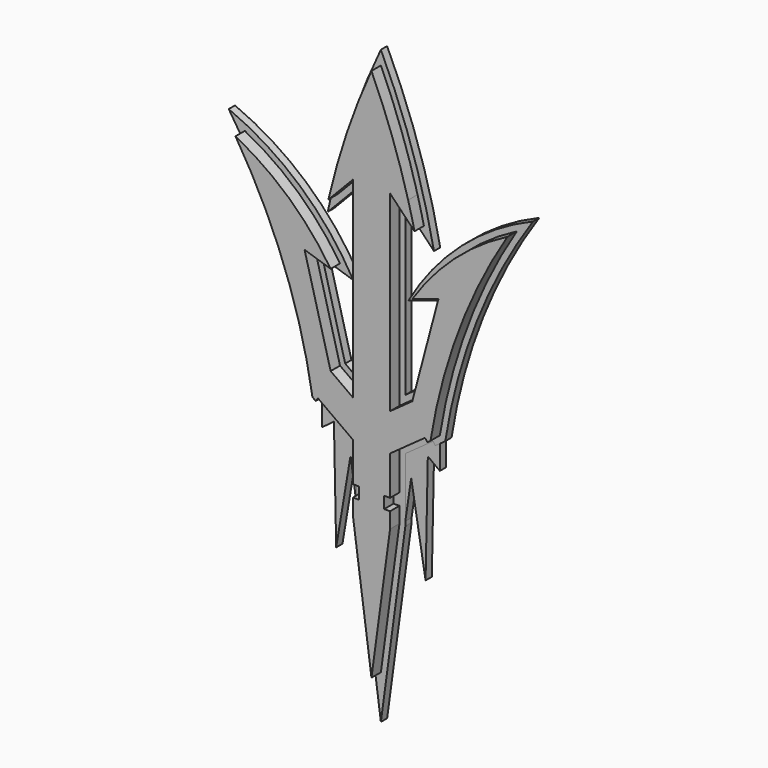
from build123d import *

# Parameters (mm, degrees)
F0_W     = 9.5
F0_H     = 3
F0_W_2   = 4.75
F0_H_2   = 6.5
F0_W_3   = 6.5
F1_DEPTH = 5
F3_DEPTH = 2
F5_DEPTH = 2


with BuildPart() as f1:
    # F0 (on Front) → F1 (new body)
    with BuildSketch(Plane.XZ):
        Polygon((4.75, -32.75), (4.75, -31.75), (0, -31.75), (-4.75, -31.75), (-4.75, -32.75), align=None)
        Polygon((0, -31.75), (4.75, -31.75), (4.75, -26.75), (4.75, -17.25), (4.75, 25.25), (0, 25.25), (-4.75, 25.25), (-4.75, -17.25), (-4.75, -26.75), (-4.75, -31.75), align=None)
        with BuildLine():
            Line((4.75, -17.25), (4.75, -26.75))
            Line((4.75, -26.75), (13.6785707143, -20.325))
            Line((13.6785707143, -20.325), (14.2626616234, -21.1366882468))
            Line((14.2626616234, -21.1366882468), (15.0743498701, -20.5525973377))
            ThreePointArc((15.0743498701, -20.5525973377), (22.2760836347, 6.5903692937), (34.75, 31.75))
            ThreePointArc((34.75, 31.75), (21.1663739273, 22.3753288761), (10.4318177273, 9.8386363636))
            Line((10.4318177273, 9.8386363636), (17.0997445143, 11.9690711462))
            Line((17.0997445143, 11.9690711462), (10.4318177273, -13.1613636364))
            Line((10.4318177273, -13.1613636364), (4.75, -17.25))
        make_face()
        with Locations((0, -34.25)):
            Rectangle(F0_W, F0_H)
        Polygon((4.75, -36.75), (4.75, -35.75), (-4.75, -35.75), (-4.75, -36.75), (-3.25, -36.75), (3.25, -36.75), align=None)
        with BuildLine():
            Line((-13.6785707143, -20.325), (-4.75, -26.75))
            Line((-4.75, -26.75), (-4.75, -17.25))
            Line((-4.75, -17.25), (-10.4318177273, -13.1613636364))
            Line((-10.4318177273, -13.1613636364), (-17.0997445143, 11.9690711462))
            Line((-17.0997445143, 11.9690711462), (-10.4318177273, 9.8386363636))
            ThreePointArc((-10.4318177273, 9.8386363636), (-21.1663739273, 22.3753288761), (-34.75, 31.75))
            ThreePointArc((-34.75, 31.75), (-22.2760836347, 6.5903692937), (-15.0743498701, -20.5525973377))
            Line((-15.0743498701, -20.5525973377), (-14.2626616234, -21.1366882468))
            Line((-14.2626616234, -21.1366882468), (-13.6785707143, -20.325))
        make_face()
        with Locations((2.375, 28.5)):
            Rectangle(F0_W_2, F0_H_2)
        Polygon((8.8, 31.75), (4.75, 31.75), (11, 25.25), align=None)
        Polygon((0, 31.75), (4.75, 31.75), (8.8, 31.75), (0, 57.75), align=None)
        with Locations((-2.375, 28.5)):
            Rectangle(F0_W_2, F0_H_2)
        with BuildLine():
            Line((8.8, 31.75), (11, 25.25))
            ThreePointArc((11, 25.25), (10.2159514871, 28.5079487405), (9.3685639152, 31.75))
            Line((9.3685639152, 31.75), (8.8, 31.75))
        make_face()
        with Locations((0, -38.25)):
            Rectangle(F0_W_3, F0_H)
        Polygon((-4.75, 31.75), (0, 31.75), (0, 57.75), (-11, 25.25), align=None)
        with BuildLine():
            Line((0, 57.75), (8.8, 31.75))
            Line((8.8, 31.75), (9.3685639152, 31.75))
            ThreePointArc((9.3685639152, 31.75), (5.207479083, 44.9385232965), (0, 57.75))
        make_face()
        Polygon((4.75, -39.75), (3.25, -39.75), (-3.25, -39.75), (-4.75, -39.75), (-4.75, -40.75), (4.75, -40.75), align=None)
        with BuildLine():
            ThreePointArc((0, 57.75), (-6.3126627605, 41.7750550882), (-11, 25.25))
            Line((-11, 25.25), (0, 57.75))
        make_face()
        Polygon((4.75, -43.75), (4.75, -40.75), (-4.75, -40.75), (-4.75, -43.75), (0, -43.75), align=None)
        Polygon((0, -78.75), (4.75, -43.75), (0, -43.75), align=None)
        Polygon((0, -43.75), (-4.75, -43.75), (0, -78.75), align=None)
    extrude(amount=F1_DEPTH)


with BuildPart() as f3:
    # F2 (on face) → F3 (new body)
    with BuildSketch(Plane(origin=(0, 0, 0), x_dir=(-1, 0, 0), z_dir=(0, 1, 0))):
        Polygon((15.0743498701, -28.5525973377), (15.0743498701, -20.5525973377), (14.2626616234, -21.1366882468), (13.6785707143, -20.325), (4.75, -26.75), (4.75, -36.75), (3.25, -36.75), (3.25, -39.75), (4.75, -39.75), (4.75, -43.75), (0, -78.75), (1, -78.75), (7.7438349836, -32.4999243021), (11.4220166579, -54.3695688248), (11.9964974001, -26.2390598655), align=None)
    extrude(amount=-F3_DEPTH)


with BuildPart() as f3b:
    # F2 (on face) → F3, piece 2 (new body)
    with BuildSketch(Plane(origin=(0, 0, 0), x_dir=(-1, 0, 0), z_dir=(0, 1, 0))):
        Polygon((-1, -78.75), (0, -78.75), (-4.75, -43.75), (-4.75, -39.75), (-3.25, -39.75), (-3.25, -36.75), (-4.75, -36.75), (-4.75, -26.75), (-13.6785707143, -20.325), (-14.2626616234, -21.1366882468), (-15.0743498701, -20.5525973377), (-15.0743498701, -28.5525973377), (-11.9964974001, -26.2390598655), (-11.4220166579, -54.3695688248), (-7.7438349836, -32.4999243021), align=None)
    extrude(amount=-F3_DEPTH)


with BuildPart() as f5:
    # F4 (on face) → F5 (new body)
    with BuildSketch(Plane(origin=(0, 0, 0), x_dir=(-1, 0, 0), z_dir=(0, 1, 0))):
        with BuildLine():
            Line((9.1197276527, -12.2575435817), (6.25, -14.3225997658))
            Line((6.25, -14.3225997658), (6.25, 28.0258373444))
            Line((6.25, 28.0258373444), (13.5709714754, 20.4120270099))
            ThreePointArc((13.5709714754, 20.4120270099), (8.0601511253, 41.2813035717), (0, 61.3045353033))
            ThreePointArc((0, 61.3045353033), (-8.0601511253, 41.2813035717), (-13.5709714754, 20.4120270099))
            Line((-13.5709714754, 20.4120270099), (-6.25, 28.0258373444))
            Line((-6.25, 28.0258373444), (-6.25, -14.3225997658))
            Line((-6.25, -14.3225997658), (-9.1197276527, -12.2575435817))
            Line((-9.1197276527, -12.2575435817), (-14.9475706012, 9.7067388435))
            Line((-14.9475706012, 9.7067388435), (-7.0573343808, 7.185770299))
            ThreePointArc((-7.0573343808, 7.185770299), (-20.623685191, 23.9014967836), (-38.8766030738, 35.3160653244))
            ThreePointArc((-38.8766030738, 35.3160653244), (-24.5064831966, 8.2050547659), (-16.4583681212, -21.4046578724))
            Line((-16.4583681212, -21.4046578724), (-13.9212656169, -23.2303569805))
            Line((-13.9212656169, -23.2303569805), (-13.3371747078, -22.4186687338))
            Line((-13.3371747078, -22.4186687338), (-6.25, -27.5186000615))
            Line((-6.25, -27.5186000615), (-6.25, -38.25))
            Line((-6.25, -38.25), (-6.25, -43.8513212997))
            Line((-6.25, -43.8513212997), (0, -89.9039528787))
            Line((0, -89.9039528787), (6.25, -43.8513212997))
            Line((6.25, -43.8513212997), (6.25, -38.25))
            Line((6.25, -38.25), (6.25, -27.5186000615))
            Line((6.25, -27.5186000615), (13.3371747078, -22.4186687338))
            Line((13.3371747078, -22.4186687338), (13.9212656169, -23.2303569805))
            Line((13.9212656169, -23.2303569805), (16.4583681212, -21.4046578724))
            ThreePointArc((16.4583681212, -21.4046578724), (24.5064831966, 8.2050547659), (38.8766030738, 35.3160653244))
            ThreePointArc((38.8766030738, 35.3160653244), (20.623685191, 23.9014967836), (7.0573343808, 7.185770299))
            Line((7.0573343808, 7.185770299), (14.9475706012, 9.7067388435))
            Line((14.9475706012, 9.7067388435), (9.1197276527, -12.2575435817))
        make_face()
        with BuildLine():
            Line((-4.75, -26.75), (-13.6785707143, -20.325))
            Line((-13.6785707143, -20.325), (-14.2626616234, -21.1366882468))
            Line((-14.2626616234, -21.1366882468), (-15.0743498701, -20.5525973377))
            ThreePointArc((-15.0743498701, -20.5525973377), (-22.2760836347, 6.5903692937), (-34.75, 31.75))
            ThreePointArc((-34.75, 31.75), (-21.1663739273, 22.3753288761), (-10.4318177273, 9.8386363636))
            Line((-10.4318177273, 9.8386363636), (-17.0997445143, 11.9690711462))
            Line((-17.0997445143, 11.9690711462), (-10.4318177273, -13.1613636364))
            Line((-10.4318177273, -13.1613636364), (-4.75, -17.25))
            Line((-4.75, -17.25), (-4.75, 31.75))
            Line((-4.75, 31.75), (-11, 25.25))
            ThreePointArc((-11, 25.25), (-6.3126627605, 41.7750550882), (0, 57.75))
            ThreePointArc((0, 57.75), (6.3126627605, 41.7750550882), (11, 25.25))
            Line((11, 25.25), (4.75, 31.75))
            Line((4.75, 31.75), (4.75, -17.25))
            Line((4.75, -17.25), (10.4318177273, -13.1613636364))
            Line((10.4318177273, -13.1613636364), (17.0997445143, 11.9690711462))
            Line((17.0997445143, 11.9690711462), (10.4318177273, 9.8386363636))
            ThreePointArc((10.4318177273, 9.8386363636), (21.1663739273, 22.3753288761), (34.75, 31.75))
            ThreePointArc((34.75, 31.75), (22.2760836347, 6.5903692937), (15.0743498701, -20.5525973377))
            Line((15.0743498701, -20.5525973377), (14.2626616234, -21.1366882468))
            Line((14.2626616234, -21.1366882468), (13.6785707143, -20.325))
            Line((13.6785707143, -20.325), (4.75, -26.75))
            Line((4.75, -26.75), (4.75, -36.75))
            Line((4.75, -36.75), (3.25, -36.75))
            Line((3.25, -36.75), (3.25, -39.75))
            Line((3.25, -39.75), (4.75, -39.75))
            Line((4.75, -39.75), (4.75, -43.75))
            Line((4.75, -43.75), (0, -78.75))
            Line((0, -78.75), (-4.75, -43.75))
            Line((-4.75, -43.75), (-4.75, -39.75))
            Line((-4.75, -39.75), (-3.25, -39.75))
            Line((-3.25, -39.75), (-3.25, -36.75))
            Line((-3.25, -36.75), (-4.75, -36.75))
            Line((-4.75, -36.75), (-4.75, -26.75))
        make_face(mode=Mode.SUBTRACT)
    extrude(amount=-F5_DEPTH)


solid = Compound([f1.part, f3.part, f3b.part, f5.part])
